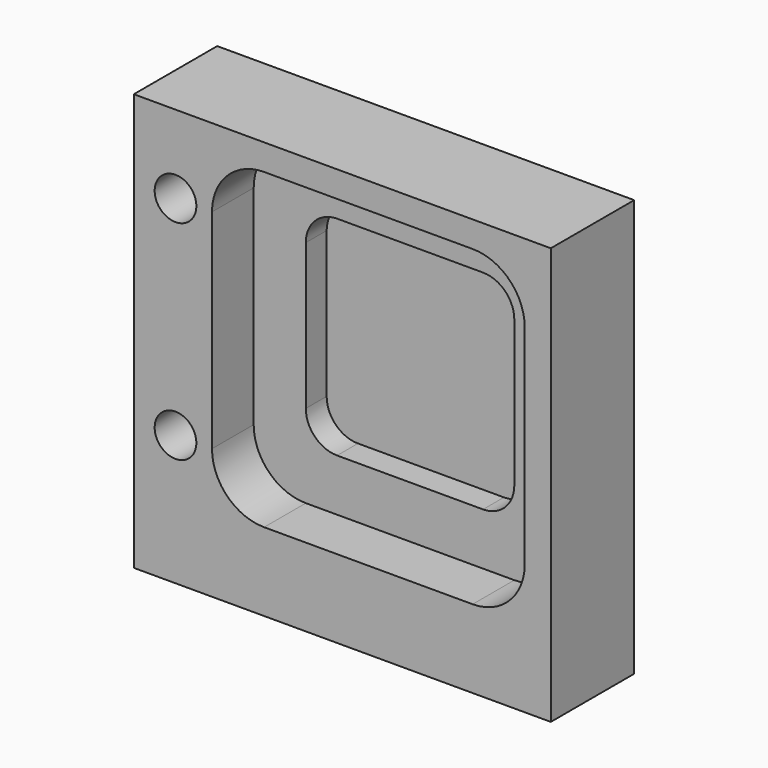
from build123d import *

# Parameters (mm, degrees)
F0_W     = 80
F0_H     = 80
F1_DEPTH = 20
F3_D     = 8
F3_DEPTH = 15
F3_TIP   = 2.4034424761
F5_DEPTH = 10
F6_DEPTH = 15


with BuildPart() as f1:
    # F0 (on Front) → F1 (new body)
    with BuildSketch(Plane.XZ):
        Rectangle(F0_W, F0_H)
    extrude(amount=F1_DEPTH)

    # F3
    with Locations(Plane.XZ.offset(20)):
        with Locations((-32, 25), (-32, -15)):
            Hole(F3_D / 2, depth=F3_DEPTH)
            with Locations((0, 0, -(F3_DEPTH + F3_TIP / 2))):  # 118° drill point
                Cone(0, F3_D / 2, F3_TIP, mode=Mode.SUBTRACT)

    # F4 (on face) → F5 (cut)
    with BuildSketch(Plane.XZ.offset(20)):
        with BuildLine():
            Line((-15, -25), (25, -25))
            ThreePointArc((25, -25), (32.0710678119, -22.0710678119), (35, -15))
            Line((35, -15), (35, 25))
            ThreePointArc((35, 25), (32.0710678119, 32.0710678119), (25, 35))
            Line((25, 35), (-15, 35))
            ThreePointArc((-15, 35), (-22.0710678119, 32.0710678119), (-25, 25))
            Line((-25, 25), (-25, -15))
            ThreePointArc((-25, -15), (-22.0710678119, -22.0710678119), (-15, -25))
        make_face()
        with BuildLine():
            ThreePointArc((25, -9), (23.2426406871, -13.2426406871), (19, -15))
            Line((19, -15), (-9, -15))
            ThreePointArc((-9, -15), (-13.2426406871, -13.2426406871), (-15, -9))
            Line((-15, -9), (-15, 19))
            ThreePointArc((-15, 19), (-13.2426406871, 23.2426406871), (-9, 25))
            Line((-9, 25), (19, 25))
            ThreePointArc((19, 25), (23.2426406871, 23.2426406871), (25, 19))
            Line((25, 19), (25, -9))
        make_face(mode=Mode.SUBTRACT)
    extrude(amount=-F5_DEPTH, mode=Mode.SUBTRACT)

    # F6 (cut): a face of the model
    f6_faces = [f1.faces().sort_by_distance(p)[0] for p in [
        (5, -20, 5),
    ]]
    extrude(f6_faces, amount=-F6_DEPTH, mode=Mode.SUBTRACT)


solid = f1.part
